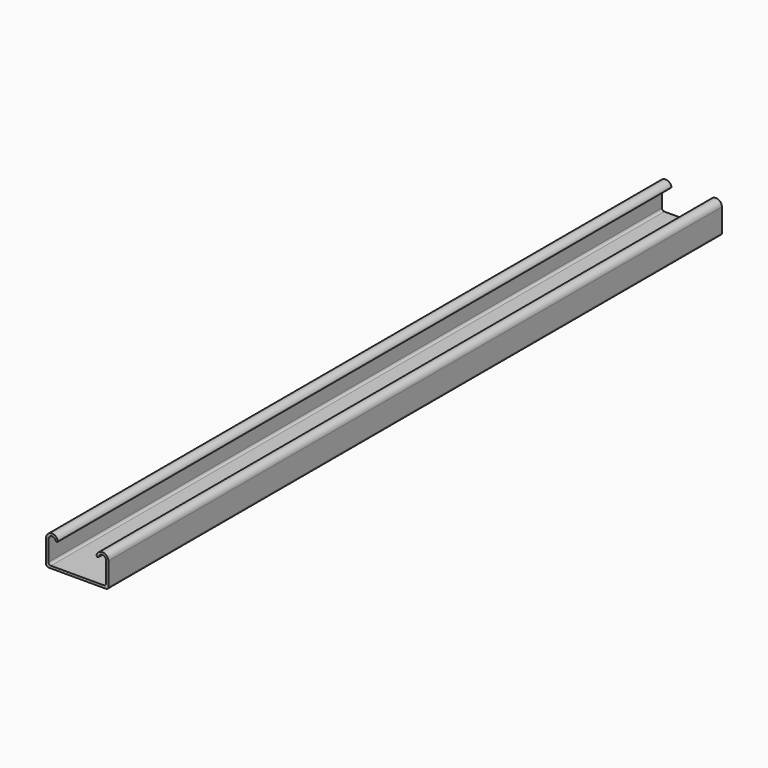
from build123d import *

# Parameters (mm, degrees)
F1_DEPTH    = 254
F2_R        = 1.5875
F3_T1_DEPTH = 511.5860222341
F3_T3_DEPTH = 513.2602424874


# Not quite as in the source:
# - a fillet or chamfer that OpenCascade refuses, or shapes differently, is made with other operations: its cross-section is extruded or revolved along the edge and cut away or added


with BuildPart() as f1:
    # F0 (on Front) → F1 (new body, symmetric)
    with BuildSketch(Plane.XZ):
        with BuildLine():
            Line((0, 16.6624), (0, 0))
            Line((0, 0), (41.275, 0))
            Line((41.275, 0), (41.275, 16.6624))
            ThreePointArc((41.275, 16.6624), (37.3126, 20.6248), (33.3502, 16.6624))
            Line((33.3502, 16.6624), (34.9377, 16.6624))
            ThreePointArc((34.9377, 16.6624), (37.3126, 19.0373), (39.6875, 16.6624))
            Line((39.6875, 16.6624), (39.6875, 1.5875))
            Line((39.6875, 1.5875), (1.5875, 1.5875))
            Line((1.5875, 1.5875), (1.5875, 16.6624))
            Line((1.5875, 16.6624), (0, 16.6624))
        make_face()
        with BuildLine():
            ThreePointArc((7.9248, 16.6624), (3.9624, 20.6248), (0, 16.6624))
            Line((0, 16.6624), (1.5875, 16.6624))
            ThreePointArc((1.5875, 16.6624), (3.9624, 19.0373), (6.3373, 16.6624))
            Line((6.3373, 16.6624), (7.9248, 16.6624))
        make_face()
    extrude(amount=F1_DEPTH, both=True)

    # F2
    f2_edges = [f1.edges().sort_by_distance(p)[0] for p in [
        (0, 0, 0),
        (41.275, 0, 0),
        (39.6875, 0, 1.5875),
        (1.5875, 0, 1.5875),
    ]]
    fillet(f2_edges, radius=F2_R)

    # F3: fillet of radius 0.8255 on 4 edges, made by hand

    # F3_s2 → F3_t1 (cut)
    with BuildSketch(Plane.XZ.offset(-255.793011117)):
        with BuildLine():
            ThreePointArc((34.2204955532, 16.6624), (34.723327211, 16.8332164322), (35.0180621764, 17.2749734127))
            ThreePointArc((35.0180621764, 17.2749734127), (34.957876249, 16.9713110978), (34.9377, 16.6624))
            Line((34.9377, 16.6624), (34.2204955532, 16.6624))
        make_face()
        with BuildLine():
            ThreePointArc((7.0545044468, 16.6624), (6.551672789, 16.8332164322), (6.2569378236, 17.2749734127))
            ThreePointArc((6.2569378236, 17.2749734127), (6.317123751, 16.9713110978), (6.3373, 16.6624))
            Line((6.3373, 16.6624), (7.0545044468, 16.6624))
        make_face()
    extrude(amount=F3_T1_DEPTH, mode=Mode.SUBTRACT)

    # F3_s4 → F3_t3 (cut)
    with BuildSketch(Plane.XZ.offset(-256.6301212437)):
        with BuildLine():
            ThreePointArc((33.4898635929, 17.7051368421), (33.6302261346, 16.9868405041), (34.2862670111, 16.6624))
            Line((34.2862670111, 16.6624), (33.3502, 16.6624))
            ThreePointArc((33.3502, 16.6624), (33.385271105, 17.1884242487), (33.4898635929, 17.7051368421))
        make_face()
        with BuildLine():
            ThreePointArc((7.7851364071, 17.7051368421), (7.6447738654, 16.9868405041), (6.9887329889, 16.6624))
            Line((6.9887329889, 16.6624), (7.9248, 16.6624))
            ThreePointArc((7.9248, 16.6624), (7.889728895, 17.1884242487), (7.7851364071, 17.7051368421))
        make_face()
    extrude(amount=F3_T3_DEPTH, mode=Mode.SUBTRACT)


solid = f1.part
